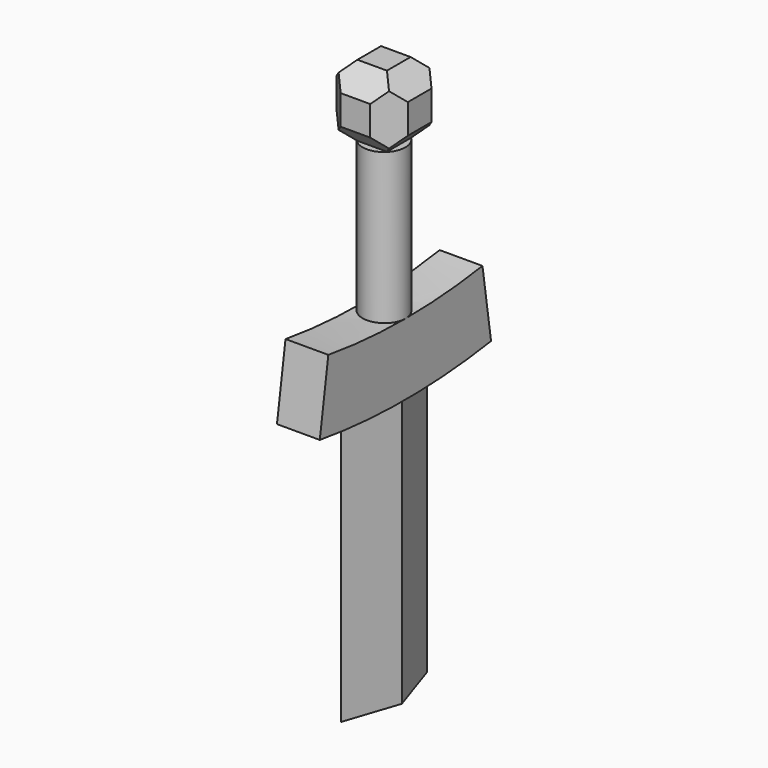
from build123d import *

# Parameters (mm, degrees)
F0_R      = 6.35
F1_DEPTH  = 1.5875
F2_R      = 6.35
F2_R_2    = 5.715
F3_DEPTH  = 0.79375
F5_DEPTH  = 12.7
F7_DEPTH  = 0.762
F8_W      = 0.762
F8_H      = 7.62
F11_DEPTH = 2.54
F13_DEPTH = 25.4
F15_DEPTH = 7.621
F16_W     = 24.9132402241
F16_H     = 7.0053068921
F17_DEPTH = 12.7


# Not quite as in the source:
# - a feature names something its author has since deleted; it is built from what else it names


with BuildPart() as f1:
    # F0 (on Top) → F1 (new body)
    with BuildSketch(Plane.XY):
        Circle(F0_R)
    extrude(amount=F1_DEPTH)

    # F2 (on face) → F3 (join)
    with BuildSketch(Plane.XY.offset(1.5875)):
        Circle(F2_R)
        Circle(F2_R_2, mode=Mode.SUBTRACT)
        with BuildLine():
            add(Edge.make_bspline(
                [(2.9683180619, -0.4757996358), (2.843389073, -0.4786165828), (2.7050840949, -0.5086647904), (2.5873180619, -0.5161623703)],
                knots=[0.409339872, 0.409339872, 0.409339872, 0.409339872, 0.4280905329, 0.4280905329, 0.4280905329, 0.4280905329], degree=3))
            add(Edge.make_bspline(
                [(2.5873180619, -0.5161623703), (2.4915986751, -0.5222563495), (2.3352190965, -0.5054979102), (2.1335509903, -0.5700528844), (1.886210527, -0.6696578597), (1.7267290127, -0.8313152566), (1.6781527788, -1.0212940602), (1.5990320903, -1.1897273451), (1.6464089719, -1.2957044031), (1.5599711629, -1.4279363767), (1.5051186748, -1.5717824942), (1.450980873, -1.6442395094), (1.453928646, -1.7165163565), (1.513053832, -1.7807591134), (1.5434308822, -1.8303185726), (1.576198943, -1.9162350186), (1.5055990352, -1.9919946196), (1.4668165836, -2.0222182295), (1.4097694676, -2.0618705924), (1.4071401198, -2.0762813928), (1.407019912, -2.0936682429), (1.4054410858, -2.1159814671), (1.4256709316, -2.1343567811), (1.4482180902, -2.1520382899), (1.5329915239, -2.3033090939), (1.6303822196, -2.3814989965), (1.5935632797, -2.4623744081), (1.5348318369, -2.4983128964), (1.4776982069, -2.5441298885), (1.455742429, -2.5511454253), (1.4798178263, -2.5621456444), (1.4948688399, -2.5838079134), (1.5251861888, -2.6046329809), (1.4935773749, -2.6345303194), (1.4713860455, -2.6758526458), (1.4221955197, -2.712885243), (1.3936565716, -2.7915463541), (1.4945229102, -2.8204202545), (1.6288484983, -2.8640100665), (1.7728549214, -2.853346582), (1.9116412442, -2.8061555548), (2.0472725737, -2.770170597), (2.2043787565, -2.7459265468), (2.3033355203, -2.7551939211), (2.3339263508, -2.8073911697), (2.353376687, -2.8775353249), (2.3257401171, -2.9468505336), (2.3037614678, -3.0393999235), (2.1498886548, -3.0666616669), (2.0714102198, -3.0904863786), (1.9727168734, -3.1134789891), (1.7843150368, -3.140535518), (1.6436061221, -3.1389483141), (1.5234236482, -3.1049579495), (1.4521295971, -3.0857303745), (1.4124230671, -3.1305535957), (1.4949213438, -3.1891776378), (1.5227733168, -3.2831967132), (1.4841449535, -3.3566867509), (1.4775180681, -3.4518910587), (1.4608440665, -3.566216612), (1.549729833, -3.6446920788), (1.8994677395, -3.667719288), (2.0536618712, -3.5673701183), (2.086254186, -3.5448411945)],
                knots=[0.4280905329, 0.4280905329, 0.4280905329, 0.4280905329, 0.4433309355, 0.457101701, 0.472691433, 0.4868290747, 0.5002944463, 0.5129981027, 0.5225928523, 0.5342722129, 0.5463608736, 0.5552384945, 0.5629095325, 0.5716491532, 0.5791344546, 0.5877870081, 0.596979654, 0.6042024841, 0.6118646332, 0.6153039035, 0.6192184677, 0.6236552276, 0.6283160232, 0.6333712575, 0.6459326281, 0.6564149698, 0.6642919572, 0.6725026939, 0.6807518007, 0.684185616, 0.6882292359, 0.6934969149, 0.6985507014, 0.7041050254, 0.7107743014, 0.7183805652, 0.7259377484, 0.7347425449, 0.7463542944, 0.7577985049, 0.7693099164, 0.780784325, 0.7929687375, 0.8020678672, 0.8090716285, 0.8170400104, 0.8252507415, 0.834055538, 0.845515778, 0.8543322878, 0.8638427207, 0.8770648317, 0.8886457092, 0.899333178, 0.9072373981, 0.9129559403, 0.9218532611, 0.9311181429, 0.9395692705, 0.9490169241, 0.9588418554, 0.9683094215, 0.9861710617, 1, 1, 1, 1], degree=3))
            add(Edge.make_bspline(
                [(2.086254186, -3.5448411945), (2.1011047055, -3.5345760071), (2.1201833918, -3.5199789546), (2.2133903471, -3.4742318908), (2.3333214203, -3.4513666992), (2.4607568415, -3.4062321353), (2.6387662736, -3.3641035898), (2.7563669715, -3.3392389367), (2.8861628847, -3.3278317932), (2.9202917573, -3.1985664964), (2.9487510475, -3.0806210272), (2.9453740986, -2.8830592898), (2.9475003966, -2.7801627945), (3.0024526725, -2.634440086), (3.0665778639, -2.4862895949), (3.1278419801, -2.4963691695), (3.2148748542, -2.5174044884), (3.2670738053, -2.6357726537), (3.300079047, -2.7251932385), (3.4018745991, -2.7381242004), (3.5380519165, -2.7491446387), (3.665083714, -2.6861808801), (3.7982425029, -2.6394629665), (3.9059135519, -2.5530868531), (4.0451426633, -2.4694400612), (4.1647565761, -2.2912192854), (4.2419872332, -2.1073390896), (4.3180155802, -1.9393229235), (4.3188699133, -1.6520894893), (4.249875342, -1.4134518517), (4.1905089106, -1.1973159772), (4.0374858266, -0.958444693), (3.8993633614, -0.7738144821), (3.5856153955, -0.5701629325), (3.286341595, -0.5131462763), (3.0825055806, -0.4732248916), (2.9683180619, -0.4757996358)],
                knots=[0, 0, 0, 0, 0.0063010841, 0.0157194351, 0.0263949763, 0.0376453369, 0.0505479911, 0.0613137498, 0.071480671, 0.0817330319, 0.0926649823, 0.1059401058, 0.1157236868, 0.1278653869, 0.1394743491, 0.1461226676, 0.1548216508, 0.1655548739, 0.1745318922, 0.1836808664, 0.1948523405, 0.2062053504, 0.2175283386, 0.2286731355, 0.2407902953, 0.2547394428, 0.2682405406, 0.2811697816, 0.2972000982, 0.3123569589, 0.3266907485, 0.3425591711, 0.3572627122, 0.3754272219, 0.3922014044, 0.409339872, 0.409339872, 0.409339872, 0.409339872], degree=3))
        make_face()
        with BuildLine():
            add(Edge.make_bspline(
                [(1.6971518053, -1.7743168864), (1.6817021758, -1.7925924294), (1.6769970047, -1.8625052871), (1.729693431, -1.9463010045), (1.7845566819, -2.0039238946), (1.7796195304, -2.0789246327), (1.7537680377, -2.1257688745), (1.8014879536, -2.2093126279), (1.9177102455, -2.1779080217), (1.965096075, -2.0707704095), (1.9605129281, -1.9856512165), (1.9580791022, -1.8944092615), (1.8839995072, -1.8212095405), (1.8202543113, -1.7813944492), (1.7573140981, -1.749016499), (1.7102858438, -1.7587804824), (1.6971518053, -1.7743168864)],
                knots=[0, 0, 0, 0, 0.0723902032, 0.1521785163, 0.2220894047, 0.2876074386, 0.3444825904, 0.4130481958, 0.4920977039, 0.5756332962, 0.6493011321, 0.723443126, 0.8024927151, 0.8724037498, 0.9384596426, 1, 1, 1, 1], degree=3))
        make_face(mode=Mode.SUBTRACT)
        with BuildLine():
            add(Edge.make_bspline(
                [(-2.4699478998, -0.4572949838), (-2.5708650863, -0.4563367572), (-2.7369839982, -0.4424518124), (-2.9380629804, -0.5061475005), (-3.1861355879, -0.6061766595), (-3.3454329941, -0.7677273894), (-3.3940542763, -0.9577322927), (-3.4731643105, -1.1261594047), (-3.4257896257, -1.2321377355), (-3.5122267839, -1.364369332), (-3.5670794532, -1.5082155546), (-3.6212172198, -1.5806725493), (-3.6182694543, -1.6529494008), (-3.5591442662, -1.7171921565), (-3.5287672166, -1.766751616), (-3.4959991555, -1.8526680619), (-3.5665990634, -1.9284276629), (-3.605381515, -1.9586512728), (-3.662428631, -1.9983036357), (-3.6650579788, -2.0127144361), (-3.6651781866, -2.0301012863), (-3.6667570128, -2.0524145104), (-3.646527167, -2.0707898244), (-3.6239800084, -2.0884713333), (-3.5392065747, -2.2397421372), (-3.441815879, -2.3179320399), (-3.4786348188, -2.3988074514), (-3.5373662617, -2.4347459398), (-3.5944998917, -2.4805629318), (-3.6164556696, -2.4875784687), (-3.5923802723, -2.4985786877), (-3.5773292587, -2.5202409567), (-3.5470119098, -2.5410660242), (-3.5786207237, -2.5709633628), (-3.600812053, -2.6122856891), (-3.6500025789, -2.6493182863), (-3.678541527, -2.7279793974), (-3.5776751884, -2.7568532979), (-3.4433496003, -2.8004431099), (-3.2993431772, -2.7897796254), (-3.1605568544, -2.7425885981), (-3.0249255249, -2.7066036403), (-2.8678193421, -2.6823595901), (-2.7688625783, -2.6916269644), (-2.7382717478, -2.743824213), (-2.7188214116, -2.8139683683), (-2.7464579815, -2.8832835769), (-2.7684366308, -2.9758329669), (-2.9223094438, -3.0030947102), (-3.0007878788, -3.026919422), (-3.0994812252, -3.0499120324), (-3.2878830618, -3.0769685613), (-3.4285919765, -3.0753813574), (-3.5487744504, -3.0413909928), (-3.6200685015, -3.0221634179), (-3.6597750314, -3.066986639), (-3.5772767548, -3.1256106812), (-3.5494247818, -3.2196297565), (-3.5880531451, -3.2931197942), (-3.5946800305, -3.388324102), (-3.6113540321, -3.5026496554), (-3.5224682656, -3.5811251221), (-3.1727303591, -3.6041523313), (-3.0185362274, -3.5038031616), (-2.9859439126, -3.4812742379)],
                knots=[0.4276093612, 0.4276093612, 0.4276093612, 0.4276093612, 0.4432926757, 0.4570643878, 0.4726551912, 0.4867938046, 0.5002601016, 0.5129646311, 0.5225600402, 0.5342402035, 0.5463296951, 0.5552079262, 0.5628794914, 0.5716197128, 0.5791055286, 0.5877586768, 0.5969519545, 0.604175281, 0.6118379567, 0.6152774634, 0.6191922967, 0.6236293616, 0.6282904775, 0.6333460592, 0.6459082931, 0.6563913553, 0.6642688841, 0.6724801851, 0.6807298588, 0.6841639101, 0.688207808, 0.693475849, 0.6985299829, 0.7040846887, 0.710754423, 0.7183612095, 0.7259189122, 0.7347243139, 0.7463368614, 0.7577818585, 0.7692940611, 0.7807692583, 0.7929545082, 0.8020542633, 0.809058506, 0.8170274356, 0.825238731, 0.8340441327, 0.8455051603, 0.8543222761, 0.8638333627, 0.8770563824, 0.8886380559, 0.8993262592, 0.9072310226, 0.9129499578, 0.9218478901, 0.9311134087, 0.9395651171, 0.9490134201, 0.9588390266, 0.9683072434, 0.9861701112, 1, 1, 1, 1], degree=3))
            add(Edge.make_bspline(
                [(-2.9859439126, -3.4812742379), (-2.9710933931, -3.4710090504), (-2.9520147068, -3.456411998), (-2.8588077515, -3.4106649341), (-2.7388766783, -3.3877997425), (-2.6114412571, -3.3426651787), (-2.433431825, -3.3005366331), (-2.3158311271, -3.27567198), (-2.1860352139, -3.2642648366), (-2.1519063413, -3.1349995397), (-2.1234470511, -3.0170540705), (-2.1268239999, -2.8194923331), (-2.1246977019, -2.7165958378), (-2.0697454261, -2.5708731293), (-2.0056202347, -2.4227226382), (-1.9443561185, -2.4328022129), (-1.8573232444, -2.4538375317), (-1.8051242933, -2.5722056971), (-1.7721190516, -2.6616262819), (-1.6703234995, -2.6745572438), (-1.5341461821, -2.685577682), (-1.4071143845, -2.6226139237), (-1.2739555958, -2.5758960088), (-1.1662845461, -2.4895199003), (-1.0270554378, -2.4058730873), (-0.9074415115, -2.2276524028), (-0.830210904, -2.0437718725), (-0.7541823669, -1.8757569873), (-0.753328888, -1.5885177996), (-0.8223203653, -1.3499010029), (-0.8816979637, -1.1336899083), (-1.0346766678, -0.8951175642), (-1.1729684536, -0.7093468208), (-1.4859704608, -0.5107200004), (-1.7852685997, -0.4361256058), (-1.9796795123, -0.4407184694), (-2.0889478998, -0.4452950088)],
                knots=[0, 0, 0, 0, 0.0063015172, 0.0157205155, 0.0263967904, 0.0376479243, 0.0505514652, 0.0613179639, 0.0714855839, 0.0817386494, 0.0926713511, 0.1059473871, 0.1157316405, 0.1278741751, 0.1394839351, 0.1461327105, 0.1548322917, 0.1655662524, 0.1745438878, 0.1836934908, 0.1948657327, 0.2062195229, 0.2175432893, 0.2286888521, 0.2408068447, 0.254756951, 0.2682589767, 0.2811891063, 0.2972205247, 0.3123784271, 0.3267132019, 0.3425827151, 0.3572872668, 0.3754530249, 0.3922283603, 0.4089050235, 0.4089050235, 0.4089050235, 0.4089050235], degree=3))
            add(Edge.make_bspline(
                [(-2.0889478998, -0.4452950088), (-2.2115019627, -0.4504279985), (-2.3495913807, -0.4584377902), (-2.4699478998, -0.4572949838)],
                knots=[0.4089050235, 0.4089050235, 0.4089050235, 0.4089050235, 0.4276093612, 0.4276093612, 0.4276093612, 0.4276093612], degree=3))
        make_face()
        with BuildLine():
            add(Edge.make_bspline(
                [(-3.3750462933, -1.7107499298), (-3.3904959228, -1.7290254728), (-3.3952010939, -1.7989383304), (-3.3425046676, -1.8827340479), (-3.2876414167, -1.940356938), (-3.2925785682, -2.015357676), (-3.3184300609, -2.0622019178), (-3.270710145, -2.1457456712), (-3.1544878531, -2.114341065), (-3.1071020236, -2.0072034528), (-3.1116851705, -1.9220842599), (-3.1141189964, -1.8308423049), (-3.1881985914, -1.7576425838), (-3.2519437873, -1.7178274925), (-3.3148840005, -1.6854495423), (-3.3619122548, -1.6952135257), (-3.3750462933, -1.7107499298)],
                knots=[0, 0, 0, 0, 0.0723902032, 0.1521785163, 0.2220894047, 0.2876074386, 0.3444825904, 0.4130481958, 0.4920977039, 0.5756332962, 0.6493011321, 0.723443126, 0.8024927151, 0.8724037498, 0.9384596426, 1, 1, 1, 1], degree=3))
        make_face(mode=Mode.SUBTRACT)
        with BuildLine():
            add(Edge.make_bspline(
                [(-2.0889478998, -0.4452950088), (-2.2115019627, -0.4504279985), (-2.3495913807, -0.4584377902), (-2.4699478998, -0.4572949838)],
                knots=[0.4089050235, 0.4089050235, 0.4089050235, 0.4089050235, 0.4276093612, 0.4276093612, 0.4276093612, 0.4276093612], degree=3))
            Line((-2.0889478998, -0.4452950088), (-2.0889478998, 3.3454788989))
            Line((-2.0889478998, 3.3454788989), (2.5873180619, 3.3454788989))
            Line((2.5873180619, 3.3454788989), (2.5873180619, -0.5161623703))
            add(Edge.make_bspline(
                [(2.9683180619, -0.4757996358), (2.843389073, -0.4786165828), (2.7050840949, -0.5086647904), (2.5873180619, -0.5161623703)],
                knots=[0.409339872, 0.409339872, 0.409339872, 0.409339872, 0.4280905329, 0.4280905329, 0.4280905329, 0.4280905329], degree=3))
            Line((2.9683180619, -0.4757996358), (2.9683180619, 3.7264788989))
            Line((2.9683180619, 3.7264788989), (-2.4699478998, 3.7264788989))
            Line((-2.4699478998, 3.7264788989), (-2.4699478998, -0.4572949838))
        make_face()
        with BuildLine():
            Line((-3.550226207, -2.9001818039), (-3.550226207, -2.8240964748))
            ThreePointArc((-3.550226207, -2.8240964748), (-3.6131554429, -2.8177576011), (-3.6389924242, -2.8754873201))
            Line((-3.6389924242, -2.8754873201), (-3.550226207, -2.9001818039))
        make_face()
        with BuildLine():
            Line((-3.5515612579, -2.9365690425), (-3.6409947677, -2.9101930559))
            ThreePointArc((-3.6409947677, -2.9101930559), (-3.6144088936, -2.9743756743), (-3.550226207, -3.0009613838))
            Line((-3.550226207, -3.0009613838), (-3.5515612579, -2.9365690425))
        make_face()
        Polygon((-3.4440558991, -2.9486666899), (-3.5156634292, -2.9365690425), (-3.5175228148, -3.00363102), (-3.4440558991, -3.0129749794), align=None)
        Polygon((-3.443260084, -2.8461508919), (-3.5195409908, -2.832378028), (-3.5195409908, -2.903361572), (-3.443260084, -2.9181940481), align=None)
        Polygon((-3.3330767072, -2.8514482547), (-3.4114763728, -2.849329263), (-3.4114763728, -2.9171344358), (-3.3330767072, -2.920312807), align=None)
        Polygon((-3.3340308471, -3.0290670693), (-3.3340308471, -2.9517051298), (-3.4147564909, -2.9517051298), (-3.4147564909, -3.0172944535), align=None)
        Polygon((-3.2263969659, -3.028226085), (-3.2272379501, -2.9517051298), (-3.300395201, -2.9517051298), (-3.300395201, -3.028226085), align=None)
        Polygon((-3.2250125549, -2.8408537619), (-3.301292996, -2.849329263), (-3.301292996, -2.9192534275), (-3.2239527098, -2.9192534275), align=None)
        Polygon((-3.1221265561, -2.8121171053), (-3.195283807, -2.8314576484), (-3.195283807, -2.9155467637), (-3.1221265561, -2.8995696921), align=None)
        Polygon((-3.1212855718, -3.011408262), (-3.1204445875, -2.9365690425), (-3.1927613198, -2.9466596898), (-3.1919203355, -3.0214989092), align=None)
        Polygon((-3.005242779, -2.9836588074), (-3.0086062505, -2.9075582279), (-3.0876499257, -2.9239556752), (-3.0859684228, -3.0046810862), align=None)
        Polygon((-3.0060837633, -2.768390812), (-3.0859684228, -2.7952992823), (-3.0859684228, -2.8920017648), (-3.0060837633, -2.8692977503), align=None)
        Polygon((-2.9043358407, -2.7322324459), (-2.9766525729, -2.7549366932), (-2.9766525729, -2.859207103), (-2.9043358407, -2.8314576484), align=None)
        Polygon((-2.9758115886, -2.9744091444), (-2.9043358407, -2.9483414255), (-2.9043358407, -2.868456766), (-2.9758115886, -2.8920017648), align=None)
        with BuildLine():
            ThreePointArc((-2.8761449157, -2.9407734983), (-2.7976867204, -2.8913213797), (-2.7672707691, -2.8037081938))
            Line((-2.7672707691, -2.8037081938), (-2.8761449157, -2.8519913538))
            Line((-2.8761449157, -2.8519913538), (-2.8761449157, -2.9407734983))
        make_face()
        with BuildLine():
            ThreePointArc((-2.7748386963, -2.7717545163), (-2.8160666547, -2.7335813761), (-2.8715411789, -2.7246645186))
            Line((-2.8715411789, -2.7246645186), (-2.8715411789, -2.8146398254))
            Line((-2.8715411789, -2.8146398254), (-2.7748386963, -2.7717545163))
        make_face()
        with BuildLine():
            ThreePointArc((2.2973594023, -2.835321473), (2.2561314439, -2.7971483328), (2.2006569197, -2.7882314753))
            Line((2.2006569197, -2.7882314753), (2.2006569197, -2.878206782))
            Line((2.2006569197, -2.878206782), (2.2973594023, -2.835321473))
        make_face()
        with BuildLine():
            ThreePointArc((2.1960531829, -3.0043404549), (2.2745113782, -2.9548883364), (2.3049273295, -2.8672751505))
            Line((2.3049273295, -2.8672751505), (2.1960531829, -2.9155583104))
            Line((2.1960531829, -2.9155583104), (2.1960531829, -3.0043404549))
        make_face()
        Polygon((2.0963865099, -3.037976101), (2.1678622579, -3.0119083822), (2.1678622579, -2.9320237227), (2.0963865099, -2.9555687215), align=None)
        Polygon((2.1678622579, -2.7957994025), (2.0955455257, -2.8185036499), (2.0955455257, -2.9227740597), (2.1678622579, -2.8950246051), align=None)
        Polygon((2.0661143353, -2.8319577686), (1.9862296758, -2.858866239), (1.9862296758, -2.9555687215), (2.0661143353, -2.932864707), align=None)
        Polygon((2.0669553196, -3.047225764), (2.0635918481, -2.9711251846), (1.9845481729, -2.9875226319), (1.9862296758, -3.0682480428), align=None)
        Polygon((1.9509125268, -3.0749752186), (1.9517535111, -3.0001359992), (1.8794367788, -3.0102266464), (1.8802777631, -3.0850658659), align=None)
        Polygon((1.9500715425, -2.875684062), (1.8769142916, -2.8950246051), (1.8769142916, -2.9791137204), (1.9500715425, -2.9631366488), align=None)
        Polygon((1.8471855437, -2.9044207186), (1.7709051026, -2.9128962196), (1.7709051026, -2.9828203842), (1.8482453888, -2.9828203842), align=None)
        Polygon((1.8458011327, -3.0917930417), (1.8449601484, -3.0152720865), (1.7718028976, -3.0152720865), (1.7718028976, -3.0917930417), align=None)
        Polygon((1.7381672515, -3.092634026), (1.7381672515, -3.0152720865), (1.6574416077, -3.0152720865), (1.6574416077, -3.0808614101), align=None)
        Polygon((1.7391213914, -2.9150152113), (1.6607217258, -2.9128962196), (1.6607217258, -2.9807013925), (1.7391213914, -2.9838797636), align=None)
        Polygon((1.6289380146, -2.9097178485), (1.5526571078, -2.8959449846), (1.5526571078, -2.9669285286), (1.6289380146, -2.9817610048), align=None)
        Polygon((1.6281421995, -3.0122336466), (1.5565346694, -3.0001359992), (1.5546752838, -3.0671979766), (1.6281421995, -3.076541936), align=None)
        with BuildLine():
            Line((1.5206368407, -3.0001359992), (1.4312033309, -2.9737600125))
            ThreePointArc((1.4312033309, -2.9737600125), (1.457789205, -3.037942631), (1.5219718916, -3.0645283405))
            Line((1.5219718916, -3.0645283405), (1.5206368407, -3.0001359992))
        make_face()
        with BuildLine():
            Line((1.5219718916, -2.9637487605), (1.5219718916, -2.8876634315))
            ThreePointArc((1.5219718916, -2.8876634315), (1.4590426557, -2.8813245578), (1.4332056744, -2.9390542768))
            Line((1.4332056744, -2.9390542768), (1.5219718916, -2.9637487605))
        make_face()
    extrude(amount=F3_DEPTH)

    # F4 (on face) → F5 (join)
    with BuildSketch(Plane.XY.offset(1.5875)):
        Polygon((0.635, 0), (0, 1.905), (-0.635, 0), (0, -1.905), align=None)
    extrude(amount=F5_DEPTH)

    # F6 (on Right) → F7 (join, symmetric)
    with BuildSketch(Plane.YZ):
        with BuildLine():
            ThreePointArc((-3.81, 13.97), (0, 13.6826243153), (3.81, 13.97))
            Line((3.81, 13.97), (3.429, 16.4812624315))
            ThreePointArc((3.429, 16.4812624315), (0, 16.2226243153), (-3.429, 16.4812624315))
            Line((-3.429, 16.4812624315), (-3.81, 13.97))
        make_face()
    extrude(amount=F7_DEPTH, both=True)

    # F8 (on Right) → F9 (revolve)
    with BuildSketch(Plane.YZ):
        with Locations((0.381, 17.78)):
            Rectangle(F8_W, F8_H)
    revolve(axis=Axis((0, 0, 17.78), (0, 0, 1)))

    # F10 (on face) → F11 (join)
    with BuildSketch(Plane.XY.offset(21.59)):
        Polygon((-0.5260512242, -1.27), (0.5260512242, -1.27), (1.27, -0.5260512242), (1.27, 0.5260512242), (0.5260512242, 1.27), (-0.5260512242, 1.27), (-1.27, 0.5260512242), (-1.27, -0.5260512242), align=None)
    extrude(amount=F11_DEPTH)

    # F12 (on face) → F13 (cut)
    with BuildSketch(Plane.YZ.offset(1.27)):
        Polygon((1.27, 22.3339487758), (0.5260512242, 21.59), (1.27, 21.59), align=None)
        Polygon((-1.27, 21.59), (-0.5260512242, 21.59), (-1.27, 22.3339487758), align=None)
        Polygon((-1.27, 23.3860512242), (-0.5260512242, 24.13), (-1.27, 24.13), align=None)
        Polygon((1.27, 24.13), (0.5260512242, 24.13), (1.27, 23.3860512242), align=None)
    extrude(amount=-F13_DEPTH, mode=Mode.SUBTRACT)

    # F14 (on face) → F15 (cut, through all)
    with BuildSketch(Plane.XZ.offset(1.27)):
        Polygon((1.27, 21.59), (1.27, 22.3339487758), (0.5260512242, 21.59), align=None)
        Polygon((-1.27, 21.59), (-0.5260512242, 21.59), (-1.27, 22.3339487758), align=None)
        Polygon((-1.27, 23.3860512242), (-0.5260512242, 24.13), (-1.27, 24.13), align=None)
        Polygon((0.5260512242, 24.13), (1.27, 23.3860512242), (1.27, 24.13), align=None)
    extrude(amount=-F15_DEPTH, mode=Mode.SUBTRACT)

    # F16 (on face) → F17 (cut, symmetric)
    with BuildSketch(Plane.YZ.offset(0.762)):
        with Locations((3.815677017, 0.6096903235)):
            Rectangle(F16_W, F16_H)
    extrude(amount=F17_DEPTH, both=True, mode=Mode.SUBTRACT)


solid = f1.part
